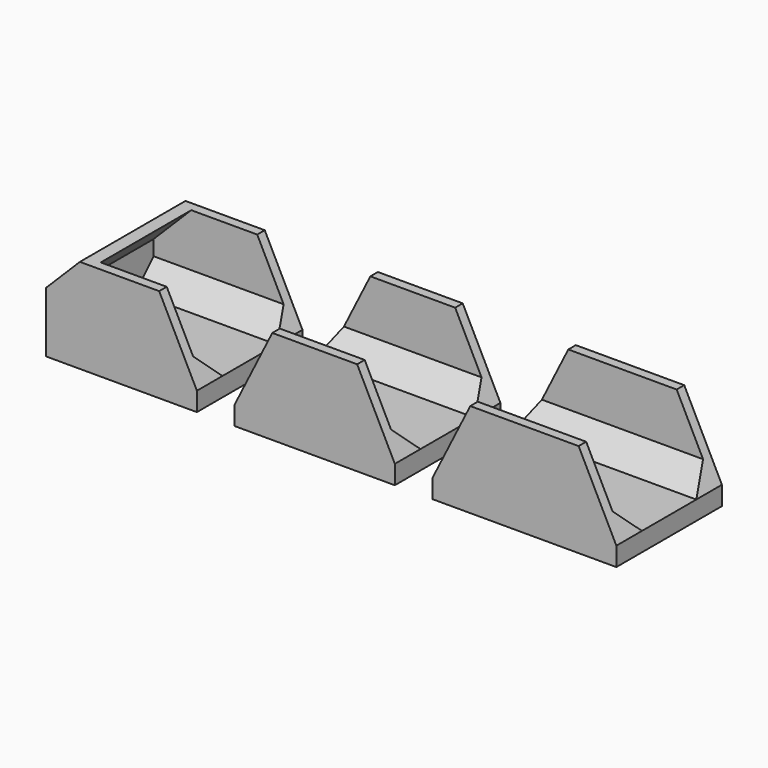
from build123d import *

# Parameters (mm, degrees)
F0_W      = 11.1125
F0_H      = 12.7
F1_DEPTH  = 11.1125
F0_W_2    = 14.2875
F0_W_3    = 18.25625
F2_DEPTH  = 9.525
F3_SIZE   = 3.81
F3_2_SIZE = 3.81
F3_3_SIZE = 3.81


# Not quite as in the source:
# - a feature names something its author has since deleted; it is built from what else it names


with BuildPart() as f1:
    # F0 (on Front) → F1 (new body, symmetric)
    with BuildSketch(Plane.XZ):
        Polygon((-46.83125, 0), (-40.48125, 0), (-40.48125, 12.7), (-46.83125, 6.35), align=None)
        Polygon((-29.36875, 0), (-23.01875, 0), (-29.36875, 12.7), align=None)
        Polygon((-48.41875, -3.175), (-46.83125, -3.175), (-46.83125, 0), (-46.83125, 6.35), (-40.48125, 12.7), (-42.7263140303, 12.7), (-48.41875, 7.0075640303), (-48.41875, 6.35), align=None)
        Polygon((-23.01875, -3.175), (-23.01875, 0), (-29.36875, 0), (-40.48125, 0), (-46.83125, 0), (-46.83125, -3.175), align=None)
        with Locations((-34.925, 6.35)):
            Rectangle(F0_W, F0_H)
    extrude(amount=F1_DEPTH, both=True)


with BuildPart() as f1b:
    # F0 (on Front) → F1, piece 2 (new body, symmetric)
    with BuildSketch(Plane.XZ):
        Polygon((-16.66875, 0), (-10.31875, 0), (-10.31875, 12.7), align=None)
        Polygon((3.96875, 0), (10.31875, 0), (3.96875, 12.7), align=None)
        Polygon((10.31875, -3.175), (10.31875, 0), (3.96875, 0), (-10.31875, 0), (-16.66875, 0), (-16.66875, -3.175), align=None)
        with Locations((-3.175, 6.35)):
            Rectangle(F0_W_2, F0_H)
    extrude(amount=F1_DEPTH, both=True)


with BuildPart() as f1c:
    # F0 (on Front) → F1, piece 3 (new body, symmetric)
    with BuildSketch(Plane.XZ):
        Polygon((23.01875, 12.7), (16.66875, 0), (23.01875, 0), align=None)
        Polygon((41.275, 0), (47.625, 0), (41.275, 12.7), align=None)
        Polygon((16.66875, 0), (16.66875, -3.175), (47.625, -3.175), (47.625, 0), (41.275, 0), (23.01875, 0), align=None)
        with Locations((32.146875, 6.35)):
            Rectangle(F0_W_3, F0_H)
    extrude(amount=F1_DEPTH, both=True)


with BuildPart() as f2_tool:
    # F0 (on Front) → F2 (new body, symmetric)
    with BuildSketch(Plane.XZ):
        Polygon((-46.83125, 0), (-40.48125, 0), (-40.48125, 12.7), (-46.83125, 6.35), align=None)
        with Locations((-34.925, 6.35)):
            Rectangle(F0_W, F0_H)
        Polygon((-29.36875, 0), (-23.01875, 0), (-29.36875, 12.7), align=None)
        with Locations((-3.175, 6.35)):
            Rectangle(F0_W_2, F0_H)
        Polygon((-16.66875, 0), (-10.31875, 0), (-10.31875, 12.7), align=None)
        Polygon((3.96875, 0), (10.31875, 0), (3.96875, 12.7), align=None)
        Polygon((23.01875, 12.7), (16.66875, 0), (23.01875, 0), align=None)
        with Locations((32.146875, 6.35)):
            Rectangle(F0_W_3, F0_H)
        Polygon((41.275, 0), (47.625, 0), (41.275, 12.7), align=None)
    extrude(amount=F2_DEPTH, both=True)


with BuildPart() as f1_1:
    add(f1.part)

    # F2: cut by f2_tool
    add(f2_tool.part, mode=Mode.SUBTRACT)

    # F3
    f3_edges = [f1_1.edges().sort_by_distance(p)[0] for p in [
        (-34.925, -9.525, 0),
        (-34.925, 9.525, 0),
    ]]
    chamfer(f3_edges, length=F3_SIZE)


with BuildPart() as f1b_1:
    add(f1b.part)

    # F2: cut by f2_tool
    add(f2_tool.part, mode=Mode.SUBTRACT)

    # F3#2
    f3_2_edges = [f1b_1.edges().sort_by_distance(p)[0] for p in [
        (-3.175, 9.525, 0),
        (-3.175, -9.525, 0),
    ]]
    chamfer(f3_2_edges, length=F3_2_SIZE)


with BuildPart() as f1c_1:
    add(f1c.part)

    # F2: cut by f2_tool
    add(f2_tool.part, mode=Mode.SUBTRACT)

    # F3#3
    f3_3_edges = [f1c_1.edges().sort_by_distance(p)[0] for p in [
        (32.146875, 9.525, 0),
        (32.146875, -9.525, 0),
    ]]
    chamfer(f3_3_edges, length=F3_3_SIZE)


solid = Compound([f1_1.part, f1b_1.part, f1c_1.part])
